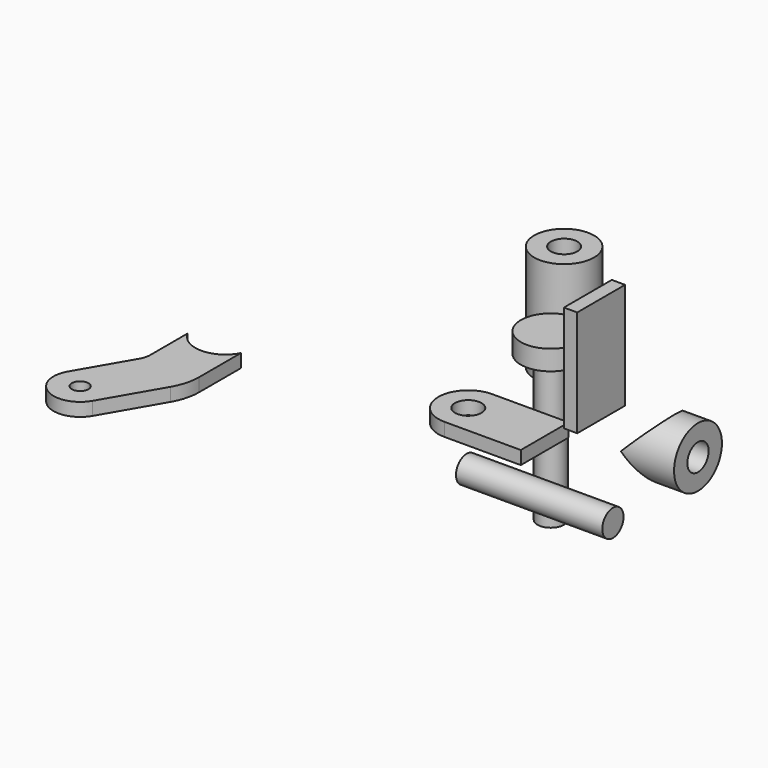
from build123d import *

# Parameters (mm, degrees)
F0_W      = 50.8
F0_H      = 28.575
F0_R      = 6.35
F1_DEPTH  = 3.175
F2_R      = 14.28749
F3_W      = 28.575
F3_H      = 50.8
F4_DEPTH  = 3.175
F5_R      = 14.2875
F5_R_2    = 6.35
F6_DEPTH  = 25.4
F7_R      = 14.2875
F8_DEPTH  = 9.525
F9_R      = 6.35
F10_DEPTH = 69.85
F11_R     = 14.2875
F12_DEPTH = 25.4
F13_R     = 6.35
F14_DEPTH = 25.4
F15_R     = 14.2875
F16_DEPTH = 14.2875
F17_R     = 6.35
F18_DEPTH = 69.85
F19_R     = 3.96875
F20_DEPTH = 3.175
F21_R     = 9.525
F22_R     = 25.4


# Not quite as in the source:
# - a fillet or chamfer is up to 0.001 mm smaller than in the source, because OpenCascade refuses the exact size


with BuildPart() as f1:
    # F0 (on Top) → F1 (new body, symmetric)
    with BuildSketch(Plane.XY):
        with Locations((-51.3317184523, -27.2989158346)):
            Rectangle(F0_W, F0_H)
        with Locations((-62.4442184523, -27.2989158346)):
            Circle(F0_R, mode=Mode.SUBTRACT)
    extrude(amount=F1_DEPTH, both=True)

    # F2 (radius 14.2875 in the source; OpenCascade refuses exactly that, so slightly less here)
    f2_edges = [f1.edges().sort_by_distance(p)[0] for p in [
        (-76.731718, -13.011416, 0),
        (-76.731718, -41.586416, 0),
    ]]
    fillet(f2_edges, radius=F2_R)


with BuildPart() as f4:
    # F3 (on Right) → F4 (new body, symmetric)
    with BuildSketch(Plane.YZ):
        with Locations((-30.0037502311, 46.1682456261)):
            Rectangle(F3_W, F3_H)
    extrude(amount=F4_DEPTH, both=True)


with BuildPart() as f6:
    # F5 (on Top) → F6 (new body, symmetric)
    with BuildSketch(Plane.XY):
        with Locations((-89.313134551, 63.5019168258)):
            Circle(F5_R)
        with Locations((-89.313134551, 63.5019168258)):
            Circle(F5_R_2, mode=Mode.SUBTRACT)
    extrude(amount=F6_DEPTH, both=True)


with BuildPart() as f8:
    # F7 (on Top) → F8 (new body)
    with BuildSketch(Plane.XY):
        with Locations((-69.5852562785, 30.8678671718)):
            Circle(F7_R)
    extrude(amount=F8_DEPTH)

    # F9 (on face) → F10 (join)
    with BuildSketch(Plane(origin=(0, 0, 0), x_dir=(1, 0, 0), z_dir=(0, 0, -1))):
        with Locations((-69.5852562785, -30.8678671718)):
            Circle(F9_R)
    extrude(amount=F10_DEPTH)


with BuildPart() as f12:
    # F11 (on Right) → F12 (new body)
    with BuildSketch(Plane.YZ):
        Circle(F11_R)
    extrude(amount=F12_DEPTH)

    # F13 (on face) → F14 (cut)
    with BuildSketch(Plane.YZ.offset(25.4)):
        Circle(F13_R)
    extrude(amount=-F14_DEPTH, mode=Mode.SUBTRACT)

    # F15 (on Top) → F16 (cut, symmetric)
    with BuildSketch(Plane.XY):
        Circle(F15_R)
    extrude(amount=F16_DEPTH, both=True, mode=Mode.SUBTRACT)


with BuildPart() as f18:
    # F17 (on Right) → F18 (new body)
    with BuildSketch(Plane.YZ):
        with Locations((-106.3271164894, 30.0037506968)):
            Circle(F17_R)
    extrude(amount=F18_DEPTH)


with BuildPart() as f20:
    # F19 (on Top) → F20 (new body, symmetric)
    with BuildSketch(Plane.XY):
        with BuildLine():
            Line((-156.3327515507, -77.3665141275), (-156.3327515507, -45.6165141275))
            ThreePointArc((-156.3327515507, -45.6165141275), (-169.0327515507, -53.3585839468), (-181.7327515507, -45.6165141275))
            Line((-181.7327515507, -45.6165141275), (-181.7327515507, -70.5400470396))
            Line((-181.7327515507, -70.5400470396), (-197.4103956987, -97.6000790939))
            ThreePointArc((-197.4103956987, -97.6000790939), (-198.6936811958, -107.2351542289), (-192.7880741077, -114.9556010713))
            ThreePointArc((-192.7880741077, -114.9556010713), (-183.1529989726, -116.2388865683), (-175.4325521302, -110.3332794802))
            Line((-175.4325521302, -110.3332794802), (-156.3327515507, -77.3665141275))
        make_face()
        with Locations((-186.4214739145, -103.966679287)):
            Circle(F19_R, mode=Mode.SUBTRACT)
    extrude(amount=F20_DEPTH, both=True)

    # F21
    f21_edges = [f20.edges().sort_by_distance(p)[0] for p in [
        (-181.732752, -70.540047, -1.5875),
        (-181.732752, -70.540047, 1.5875),
    ]]
    fillet(f21_edges, radius=F21_R)

    # F22
    f22_edges = [f20.edges().sort_by_distance(p)[0] for p in [
        (-156.332752, -77.366514, -1.5875),
        (-156.332752, -77.366514, 1.5875),
    ]]
    fillet(f22_edges, radius=F22_R)


solid = Compound([f1.part, f4.part, f6.part, f8.part, f12.part, f18.part, f20.part])
